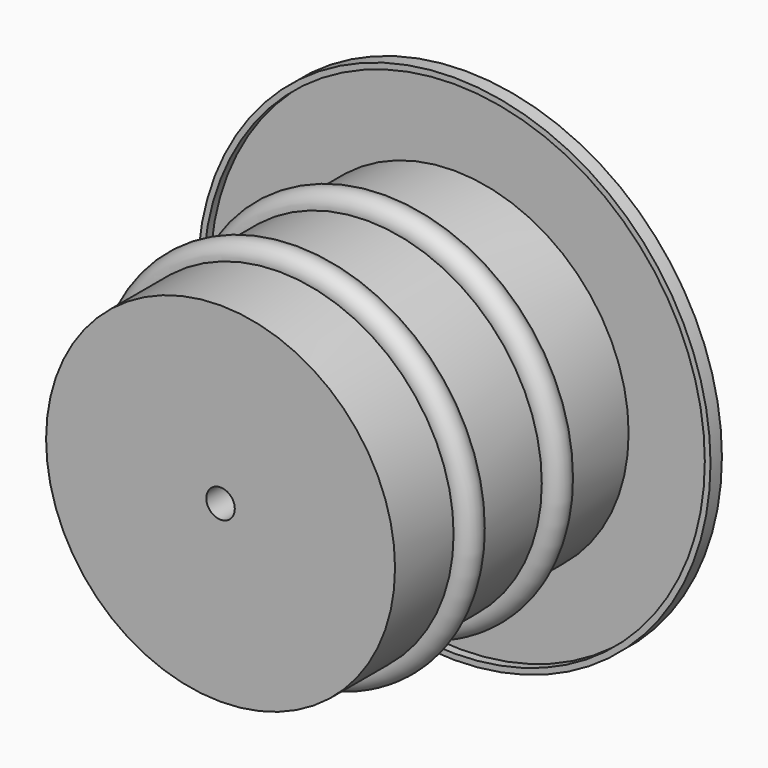
from build123d import *

# Parameters (mm, degrees)
F0_R     = 114.3
F0_R_2   = 77.7875
F1_DEPTH = 6.35
F2_DEPTH = 203.2
F3_DEPTH = 101.6
F4_R     = 6.35
F5_DEPTH = 101.601
F6_T     = -2.54
F7_DEPTH = 9.525
F8_DEPTH = 25.4
F9_R     = 6.35


# Not quite as in the source:
# - a shell that OpenCascade refuses in one call is made with other operations: the cavity is built on its own and cut out


with BuildPart() as f1:
    # F0 (on Front) → F1 (new body)
    with BuildSketch(Plane.XZ):
        Circle(F0_R)
        Circle(F0_R_2, mode=Mode.SUBTRACT)
    extrude(amount=F1_DEPTH)

    # F0 (on Front) → F2 (join)
    with BuildSketch(Plane.XZ):
        Circle(F0_R_2)
    extrude(amount=F2_DEPTH)

    # F3 (cut): a face of the model
    f3_faces = [f1.faces().sort_by_distance(p)[0] for p in [
        (0, -203.2, 0),
    ]]
    extrude(f3_faces, amount=-F3_DEPTH, mode=Mode.SUBTRACT)

    # F4 (on face) → F5 (cut, through all)
    with BuildSketch(Plane.XZ.offset(101.6)):
        Circle(F4_R)
    extrude(amount=-F5_DEPTH, mode=Mode.SUBTRACT)

    # F6: a shell. OpenCascade refuses it in one call, so the cavity is built on its own and cut out:
    # the body offset inwards by the wall thickness, plus a prism from it out through each open face.
    f6_core = offset(f1.part, amount=F6_T, kind=Kind.INTERSECTION, mode=Mode.PRIVATE)
    f6_exits = [f6_core.faces().sort_by_distance(p)[0] for p in [
        (-78.40855, -3.81, 0),
    ]]
    add(f6_core, mode=Mode.SUBTRACT)
    extrude(f6_exits, amount=-F6_T, mode=Mode.SUBTRACT)

    # F7 (add): a face of the model
    f7_faces = [f1.faces().sort_by_distance(p)[0] for p in [
        (-75.5873372503, -101.6, 0),
    ]]
    extrude(f7_faces, amount=F7_DEPTH)

    # F8 (add): a face of the model
    f8_faces = [f1.faces().sort_by_distance(p)[0] for p in [
        (-75.5873372503, -111.125, 0),
    ]]
    extrude(f8_faces, amount=F8_DEPTH)

    # F9 (on Right) → F10 (revolve)
    with BuildSketch(Plane.YZ):
        with Locations((-48.4295338392, 78.518204391)):
            Circle(F9_R)
        with Locations((-97.5811034441, 78.518204391)):
            Circle(F9_R)
    revolve(axis=Axis((0, -136.525, 0), (0, -1, 0)))


solid = f1.part
